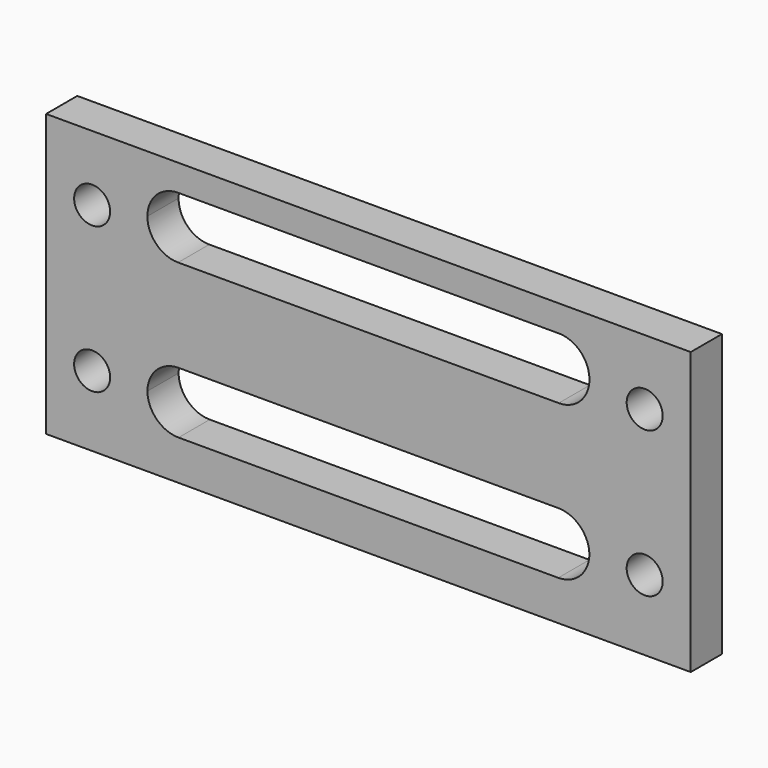
from build123d import *

# Parameters (mm, degrees)
F0_W        = 105
F0_H        = 23
F1_DEPTH    = 6.35
F2_W        = 72
F2_H        = 10
F3_DEPTH    = 25.4
F4_R        = 2.9337
F5_DEPTH    = 25.4
F6_T1_DEPTH = 6.35
F7_W        = 105
F7_H        = 23
F7_R        = 2.9335
F8_DEPTH    = 6.35
F9_W        = 72
F9_H        = 10
F10_DEPTH   = 25
F11_R       = 4.99999


# Not quite as in the source:
# - a fillet or chamfer that OpenCascade refuses, or shapes differently, is made with other operations: its cross-section is extruded or revolved along the edge and cut away or added
# - a fillet or chamfer is up to 0.001 mm smaller than in the source, because OpenCascade refuses the exact size


with BuildPart() as f1:
    # F0 (on Front) → F1 (new body)
    with BuildSketch(Plane.XZ):
        Rectangle(F0_W, F0_H)
    extrude(amount=F1_DEPTH)

    # F2 (on face) → F3 (cut)
    with BuildSketch(Plane.XZ.offset(6.35)):
        Rectangle(F2_W, F2_H)
    extrude(amount=-F3_DEPTH, mode=Mode.SUBTRACT)

    # F4 (on face) → F5 (cut)
    with BuildSketch(Plane.XZ.offset(6.35)):
        with Locations((-45, 0)):
            Circle(F4_R)
        with Locations((45, 0)):
            Circle(F4_R)
    extrude(amount=-F5_DEPTH, mode=Mode.SUBTRACT)

    # F6: fillet of radius 5.08 on 4 edges, made by hand

    # F6_s2 → F6_t1 (join)
    with BuildSketch(Plane.XZ):
        with BuildLine():
            ThreePointArc((36, 0.08), (34.5121024484, -3.5121024484), (30.92, -5))
            Line((30.92, -5), (36, -5))
            Line((36, -5), (36, 0.08))
        make_face()
        with BuildLine():
            ThreePointArc((-30.92, 5), (-34.5121024484, 3.5121024484), (-36, -0.08))
            Line((-36, -0.08), (-36, 5))
            Line((-36, 5), (-30.92, 5))
        make_face()
        with BuildLine():
            ThreePointArc((-30.92, -5), (-34.5121024484, -3.5121024484), (-36, 0.08))
            Line((-36, 0.08), (-36, -5))
            Line((-36, -5), (-30.92, -5))
        make_face()
        with BuildLine():
            ThreePointArc((36, -0.08), (34.5121024484, 3.5121024484), (30.92, 5))
            Line((30.92, 5), (36, 5))
            Line((36, 5), (36, -0.08))
        make_face()
    extrude(amount=F6_T1_DEPTH)

    # F7 (on Front) → F8 (join)
    with BuildSketch(Plane.XZ):
        with Locations((0, 22.8902743906)):
            Rectangle(F7_W, F7_H)
        with Locations((-45, 23.7624682486)):
            Circle(F7_R, mode=Mode.SUBTRACT)
        with Locations((45, 23.7624682486)):
            Circle(F7_R, mode=Mode.SUBTRACT)
    extrude(amount=F8_DEPTH)

    # F9 (on face) → F10 (cut)
    with BuildSketch(Plane.XZ.offset(6.35)):
        with Locations((0, 25.0778379703)):
            Rectangle(F9_W, F9_H)
    extrude(amount=-F10_DEPTH, mode=Mode.SUBTRACT)

    # F11 (radius 5 in the source; OpenCascade refuses exactly that, so slightly less here)
    f11_edges = [f1.edges().sort_by_distance(p)[0] for p in [
        (-36, -3.175, 20.077838),
        (36, -3.175, 20.077838),
        (36, -3.175, 30.077838),
        (-36, -3.175, 30.077838),
    ]]
    fillet(f11_edges, radius=F11_R)


solid = f1.part
